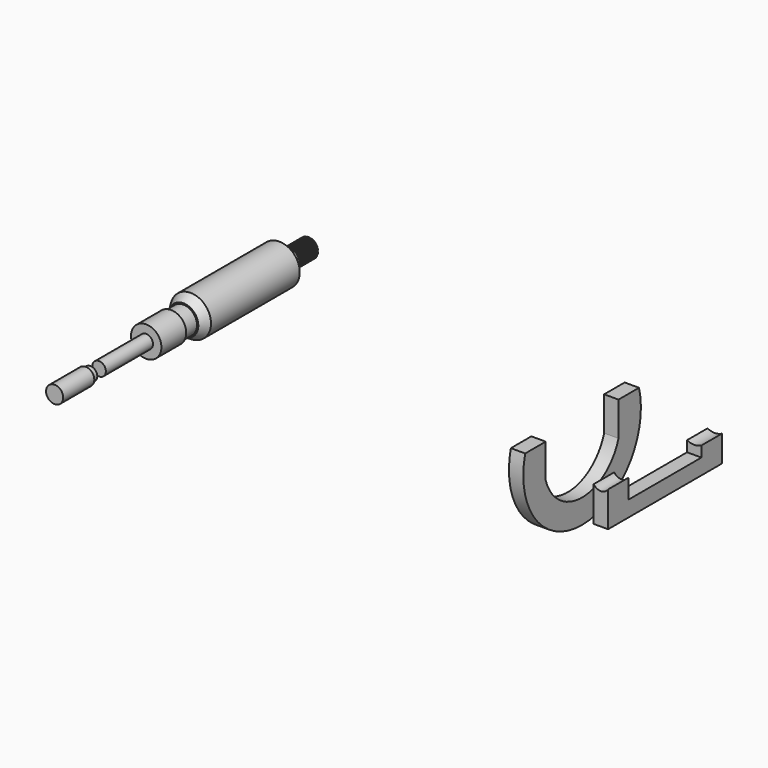
from build123d import *

# Parameters (mm, degrees)
F0_R             = 4.5
F1_DEPTH         = 17
F2_R             = 9.5
F3_DEPTH         = 56
F4_R             = 3.175
F5_DEPTH         = 33.401
F6_R             = 6.3558578776
F7_DEPTH         = 7.2136
F8_R             = 7.0975570336
F9_DEPTH         = 14.5
F12_DEPTH        = 6.7
F14_DEPTH        = 6.7
F15_SIZE2        = 4.2272698852
F15_SIZE         = 2.54
F17_DEPTH        = 11.1506
F17_COPIES_COUNT = 50
F18_R            = 3.175
F19_DEPTH        = 27.5
F19_DEPTH_BACK   = 45.466
F21_R            = 3.175
F22_DEPTH        = 2.794
F23_R            = 4.0005
F24_DEPTH        = 18.1356
F27_DEPTH        = 6.7
F28_R            = 4.0005
F29_DEPTH        = 12.827
F30_R            = 7.0975601
F31_DEPTH        = 18.9992


# Not quite as in the source:
# - a pattern or mirror of a feature is missing from the dataset's text; its kind, count and spacing are read off the source's solid


with BuildPart() as f1:
    # F0 (on Front) → F1 (new body)
    with BuildSketch(Plane.XZ):
        Circle(F0_R)
    extrude(amount=F1_DEPTH)

    # F16 (on face) → F17 (cut)
    with BuildSketch(Plane(origin=(0, 0, 0), x_dir=(-1, 0, 0), z_dir=(0, 1, 0))):
        with BuildLine():
            ThreePointArc((0.3703415092, 4.4847349048), (0.1863547671, 4.521092393), (0, 4.5))
            Line((0, 4.5), (0.1654705411, 3.9463285357))
            Line((0.1654705411, 3.9463285357), (0.3703415092, 4.4847349048))
        make_face()
    f17 = extrude(amount=-F17_DEPTH, mode=Mode.SUBTRACT)

    # F17_copies: F17 ×50 about axis
    f17_copies_axis = Axis((0, 0, 0), (0, 1, 0))
    for i in range(1, F17_COPIES_COUNT):
        add(f17.rotate(f17_copies_axis, i * 360 / F17_COPIES_COUNT), mode=Mode.SUBTRACT)


with BuildPart() as f3:
    # F2 (on face) → F3 (new body)
    with BuildSketch(Plane.XZ.offset(17)):
        Circle(F2_R)
    extrude(amount=F3_DEPTH)

    # F4 (on face) → F5 (cut)
    with BuildSketch(Plane.XZ.offset(73)):
        Circle(F4_R)
    extrude(amount=-F5_DEPTH, mode=Mode.SUBTRACT)

    # F6 (on face) → F7 (join)
    with BuildSketch(Plane.XZ.offset(73)):
        Circle(F6_R)
    extrude(amount=F7_DEPTH)

    # F8 (on face) → F9 (join)
    with BuildSketch(Plane.XZ.offset(80.2136)):
        Circle(F8_R)
    extrude(amount=F9_DEPTH)

    # F15
    f15_edges = [f3.edges().sort_by_distance(p)[0] for p in [
        (-9.5, -73, 0),
    ]]
    f15_side = f3.faces().sort_by_distance((-9.231299, -73, 0))[0]
    chamfer(f15_edges, length=F15_SIZE, length2=F15_SIZE2, reference=f15_side)


with BuildPart() as f12:
    # F11 (on offset) → F12 (new body)
    with BuildSketch(Plane.YZ.offset(127.762)):
        with BuildLine():
            ThreePointArc((-41.6519768552, -23.8150693537), (-8.4419768542, -66.7134302876), (24.7680231468, -23.8150693537))
            Line((24.7680231468, -23.8150693537), (15.3113558975, -23.8150693537))
            ThreePointArc((15.3113558975, -23.8150693537), (-8.5871562842, -53.2696518764), (-32.485668466, -23.8150693537))
            Line((-32.485668466, -23.8150693537), (-41.6519768552, -23.8150693537))
        make_face()
        with BuildLine():
            ThreePointArc((-32.485668466, -23.8150693537), (-8.5871562842, -53.2696518764), (15.3113558975, -23.8150693537))
            Line((15.3113558975, -23.8150693537), (-32.485668466, -23.8150693537))
        make_face()
    extrude(amount=F12_DEPTH)

    # F13 (on face) → F14 (cut, through all)
    with BuildSketch(Plane.YZ.offset(134.462)):
        with BuildLine():
            Line((12.795442678, -23.8150693537), (-29.6793963864, -23.8150693537))
            Line((-29.6793963864, -23.8150693537), (-29.6793963864, -39.7644422108))
            ThreePointArc((-29.6793963864, -39.7644422108), (-8.4419768542, -55.4302247587), (12.795442678, -39.7644422108))
            Line((12.795442678, -39.7644422108), (12.795442678, -23.8150693537))
        make_face()
    extrude(amount=-F14_DEPTH, mode=Mode.SUBTRACT)


with BuildPart() as f19:
    # F18 (on face) → F19 (new body, two sides)
    with BuildSketch(Plane.XZ.offset(94.7136)) as f19_sk:
        Circle(F18_R)
    extrude(amount=F19_DEPTH)
    extrude(f19_sk.sketch, amount=-F19_DEPTH_BACK)


with BuildPart() as f22:
    # F21 (on offset) → F22 (new body)
    with BuildSketch(Plane.XZ.offset(127.2136)):
        Circle(F21_R)
    extrude(amount=F22_DEPTH)


with BuildPart() as f24:
    # F23 (on face) → F24 (new body)
    with BuildSketch(Plane.XZ.offset(130.0076)):
        Circle(F23_R)
    extrude(amount=F24_DEPTH)


with BuildPart() as f27:
    # F26 (on offset) → F27 (new body)
    with BuildSketch(Plane.YZ.offset(166.466)):
        Polygon((-29.6793963864, -23.8150693537), (-41.6519768552, -23.8150693537), (-41.6519768552, -42.3790744564), (24.7680231468, -42.3790744564), (24.7680231468, -23.8150693537), (12.795442678, -23.8150693537), (12.795442678, -35.0473635634), (-29.6793963864, -35.0473635634), align=None)
    extrude(amount=F27_DEPTH)

    # F28 (on face) → F29 (cut)
    with BuildSketch(Plane.XZ.offset(41.6519768552)):
        with Locations((169.816, -23.8150693537)):
            Circle(F28_R)
    extrude(amount=-F29_DEPTH, mode=Mode.SUBTRACT)

    # F30 (on face) → F31 (cut)
    with BuildSketch(Plane.XZ.offset(-12.795442678)):
        with Locations((169.816, -23.8150693537)):
            Circle(F30_R)
    extrude(amount=-F31_DEPTH, mode=Mode.SUBTRACT)


solid = Compound([f1.part, f3.part, f12.part, f19.part, f22.part, f24.part, f27.part])
